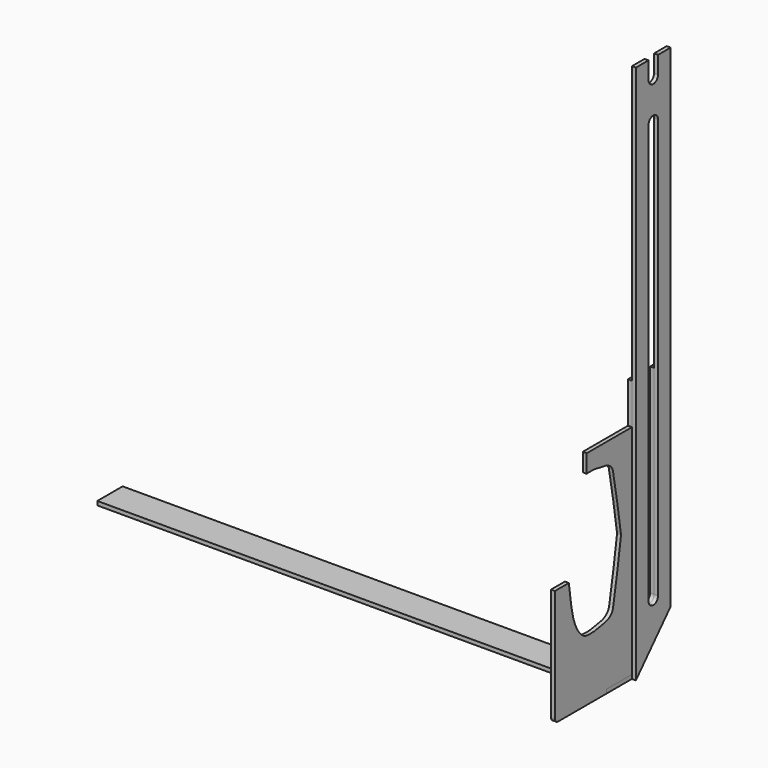
from build123d import *

# Parameters (mm, degrees)
F2_DEPTH = 12.7
F3_DEPTH = 12.7
F4_R     = 12.7
F1_W     = 101.6
F1_H     = 12.7
F5_DEPTH = 1635.125


# Not quite as in the source:
# - a feature names something its author has since deleted; it is built from what else it names


with BuildPart() as f2:
    # F1 (on offset) → F2 (new body)
    with BuildSketch(Plane.YZ.offset(304.8)):
        with BuildLine():
            Line((94.5288948266, 367.2625439401), (43.7288948266, 367.2625439401))
            Line((43.7288948266, 367.2625439401), (43.7288948266, 235.9791994095))
            Line((43.7288948266, 235.9791994095), (43.7288948266, -323.3454918831))
            Line((43.7288948266, -323.3454918831), (113.5788948266, -323.3454918831))
            Line((113.5788948266, -323.3454918831), (113.5788948266, -291.5954918831))
            ThreePointArc((113.5788948266, -291.5954918831), (100.108510645, -286.0158760647), (94.5288948266, -272.5454918831))
            Line((94.5288948266, -272.5454918831), (94.5288948266, 367.2625439401))
        make_face()
        with BuildLine():
            Line((113.5788948266, -291.5954918831), (113.5788948266, -323.3454918831))
            Line((113.5788948266, -323.3454918831), (183.4288948266, -323.3454918831))
            Line((183.4288948266, -323.3454918831), (183.4288948266, 367.2625439401))
            Line((183.4288948266, 367.2625439401), (132.6288948266, 367.2625439401))
            Line((132.6288948266, 367.2625439401), (132.6288948266, -272.5454918831))
            ThreePointArc((132.6288948266, -272.5454918831), (127.0492790082, -286.0158760647), (113.5788948266, -291.5954918831))
        make_face()
        Polygon((113.5788948266, -323.3454918831), (43.7288948266, -323.3454918831), (43.7288948266, -463.0454918831), (43.7288948266, -475.7454918831), (183.4288948266, -323.3454918831), align=None)
        with BuildLine():
            Line((43.7288948266, 1256.2625439401), (43.7288948266, 367.2625439401))
            Line((43.7288948266, 367.2625439401), (94.5288948266, 367.2625439401))
            Line((94.5288948266, 367.2625439401), (94.5288948266, 1073.6545081169))
            ThreePointArc((94.5288948266, 1073.6545081169), (100.108510645, 1087.1248922985), (113.5788948266, 1092.7045081169))
            Line((113.5788948266, 1092.7045081169), (113.5788948266, 1181.6045081169))
            ThreePointArc((113.5788948266, 1181.6045081169), (100.108510645, 1187.1841239353), (94.5288948266, 1200.6545081169))
            Line((94.5288948266, 1200.6545081169), (94.5288948266, 1256.2625439401))
            Line((94.5288948266, 1256.2625439401), (43.7288948266, 1256.2625439401))
        make_face()
        with BuildLine():
            Line((113.5788948266, 1181.6045081169), (113.5788948266, 1092.7045081169))
            ThreePointArc((113.5788948266, 1092.7045081169), (127.0492790082, 1087.1248922985), (132.6288948266, 1073.6545081169))
            Line((132.6288948266, 1073.6545081169), (132.6288948266, 367.2625439401))
            Line((132.6288948266, 367.2625439401), (183.4288948266, 367.2625439401))
            Line((183.4288948266, 367.2625439401), (183.4288948266, 1256.2625439401))
            Line((183.4288948266, 1256.2625439401), (132.6288948266, 1256.2625439401))
            Line((132.6288948266, 1256.2625439401), (132.6288948266, 1200.6545081169))
            ThreePointArc((132.6288948266, 1200.6545081169), (127.0492790082, 1187.1841239353), (113.5788948266, 1181.6045081169))
        make_face()
    extrude(amount=F2_DEPTH)


with BuildPart() as f3:
    # F1 (on offset) → F3 (new body)
    with BuildSketch(Plane.YZ.offset(304.8)):
        with BuildLine():
            Line((94.5288948266, 367.2625439401), (43.7288948266, 367.2625439401))
            Line((43.7288948266, 367.2625439401), (43.7288948266, 235.9791994095))
            Line((43.7288948266, 235.9791994095), (43.7288948266, -323.3454918831))
            Line((43.7288948266, -323.3454918831), (113.5788948266, -323.3454918831))
            Line((113.5788948266, -323.3454918831), (113.5788948266, -291.5954918831))
            ThreePointArc((113.5788948266, -291.5954918831), (100.108510645, -286.0158760647), (94.5288948266, -272.5454918831))
            Line((94.5288948266, -272.5454918831), (94.5288948266, 367.2625439401))
        make_face()
        with BuildLine():
            Line((113.5788948266, -291.5954918831), (113.5788948266, -323.3454918831))
            Line((113.5788948266, -323.3454918831), (183.4288948266, -323.3454918831))
            Line((183.4288948266, -323.3454918831), (183.4288948266, 367.2625439401))
            Line((183.4288948266, 367.2625439401), (132.6288948266, 367.2625439401))
            Line((132.6288948266, 367.2625439401), (132.6288948266, -272.5454918831))
            ThreePointArc((132.6288948266, -272.5454918831), (127.0492790082, -286.0158760647), (113.5788948266, -291.5954918831))
        make_face()
        Polygon((113.5788948266, -323.3454918831), (43.7288948266, -323.3454918831), (43.7288948266, -463.0454918831), (43.7288948266, -475.7454918831), (183.4288948266, -323.3454918831), align=None)
        with BuildLine():
            Line((43.7288948266, -323.3454918831), (43.7288948266, 235.9791994095))
            Line((43.7288948266, 235.9791994095), (-137.668, 235.9791994095))
            Line((-137.668, 235.9791994095), (-137.668, 177.8))
            add(Edge.make_bspline(
                [(-137.668, 177.8), (-126.7329989699, 179.3615885186), (-105.2927447568, 177.9606906514), (-104.7127420428, 177.4566242644), (-76.3870444308, 172.7468877699), (-53.8224361201, 169.2775097956), (-32.509347536, 153.9521162966), (-29.6589175986, 126.5444267311), (-24.1316654123, 101.7655079647), (-20.1515477066, 76.1578540031), (-15.6616591497, 50.824742265), (-11.697736498, 25.3907441448), (-7.6524561633, 0.0190908821), (-3.4145104905, -25.4546553024), (-1.1633071199, -42.1649645919), (0, -50.8)],
                knots=[0.4455893289, 0.4455893289, 0.4455893289, 0.4455893289, 0.4958311767, 0.5059382093, 0.5510171418, 0.5964071949, 0.6390826252, 0.6845795949, 0.7297371842, 0.7748161167, 0.8198950491, 0.8649377925, 0.9099805359, 0.9550232793, 1, 1, 1, 1], degree=3))
            add(Edge.make_bspline(
                [(-209.55, -101.6), (-208.6251552358, -110.5689174615), (-206.6600994581, -126.7951349357), (-202.7469529896, -152.4849572895), (-198.4813992324, -177.8058366363), (-193.5047411073, -203.4515063023), (-185.4017669459, -228.8366501901), (-172.2926489077, -254.3432279678), (-155.2398352434, -272.1810431706), (-140.6010964135, -281.8677246091), (-105.2927447568, -279.5606906514), (-104.7127420428, -279.0566242644), (-76.3870444308, -274.3468877699), (-53.8224361201, -270.8775097956), (-32.509347536, -255.5521162966), (-29.6589175986, -228.1444267311), (-24.1316654123, -203.3655079647), (-20.1515477066, -177.7578540031), (-15.6616591497, -152.424742265), (-11.697736498, -126.9907441448), (-7.6524561633, -101.6190908821), (-3.4145104905, -76.1453446976), (-1.1633071199, -59.4350354081), (0, -50.8)],
                knots=[0.0897198342, 0.0897198342, 0.0897198342, 0.0897198342, 0.1346390991, 0.1796477671, 0.2247266995, 0.269971206, 0.3159019443, 0.3636177586, 0.4065541502, 0.4455893289, 0.4958311767, 0.5059382093, 0.5510171418, 0.5964071949, 0.6390826252, 0.6845795949, 0.7297371842, 0.7748161167, 0.8198950491, 0.8649377925, 0.9099805359, 0.9550232793, 1, 1, 1, 1], degree=3))
            Line((-209.55, -101.6), (-265.2354836464, -101.6))
            Line((-265.2354836464, -101.6), (-265.2354836464, -475.7454918831))
            Line((-265.2354836464, -475.7454918831), (-57.8711051734, -475.7454918831))
            Line((-57.8711051734, -475.7454918831), (-57.8711051734, -463.0454918831))
            Line((-57.8711051734, -463.0454918831), (43.7288948266, -463.0454918831))
            Line((43.7288948266, -463.0454918831), (43.7288948266, -323.3454918831))
        make_face()
    extrude(amount=-F3_DEPTH)

    # F4
    f4_edges = [f3.edges().sort_by_distance(p)[0] for p in [
        (298.45, -265.235484, -475.745492),
        (298.45, 94.528895, 367.262544),
    ]]
    fillet(f4_edges, radius=F4_R)


with BuildPart() as f5:
    # F1 (on offset) → F5 (new body)
    with BuildSketch(Plane.YZ.offset(304.8)):
        with Locations((-7.0711051734, -469.3954918831)):
            Rectangle(F1_W, F1_H)
    extrude(amount=-F5_DEPTH)


solid = Compound([f2.part, f3.part, f5.part])
